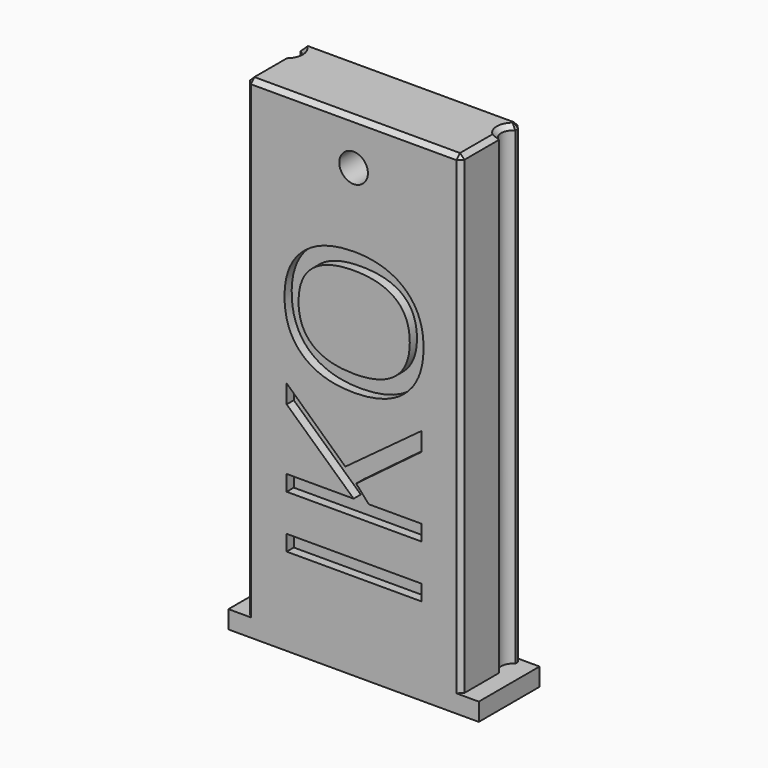
from build123d import *

# Parameters (mm, degrees)
F0_W         = 28
F0_H         = 8.5
F1_DEPTH     = 2
F3_DEPTH     = 53
F4_R         = 1.6
F5_DEPTH     = 8.501
F6_SIZE      = 0.5
F7_TEXT_SIZE = 21.1529840228
F8_DEPTH     = 1


# Not quite as in the source:
# - Text() gives the source's letters only with a copy of the font that has no kerning and outlines rounded to 1/6400 em; it was checked with that copy


with BuildPart() as f1:
    # F0 (on Top) → F1 (new body)
    with BuildSketch(Plane.XY):
        Rectangle(F0_W, F0_H)
    extrude(amount=F1_DEPTH)

    # F2 (on face) → F3 (join)
    with BuildSketch(Plane.XY.offset(2)):
        with BuildLine():
            Line((12, 4.25), (-12, 4.25))
            Line((-12, 4.25), (-12, 3.35))
            ThreePointArc((-12, 3.35), (-11.35, 2.2), (-12, 1.05))
            Line((-12, 1.05), (-12, -4.25))
            Line((-12, -4.25), (12, -4.25))
            Line((12, -4.25), (12, 1.05))
            ThreePointArc((12, 1.05), (11.35, 2.2), (12, 3.35))
            Line((12, 3.35), (12, 4.25))
        make_face()
    extrude(amount=F3_DEPTH)

    # F4 (on face) → F5 (cut, through all)
    with BuildSketch(Plane(origin=(0, 4.25, 0), x_dir=(-1, 0, 0), z_dir=(0, 1, 0))):
        with Locations((0, 50)):
            Circle(F4_R)
    extrude(amount=-F5_DEPTH, mode=Mode.SUBTRACT)

    # F6
    f6_edges = [f1.edges().sort_by_distance(p)[0] for p in [
        (12, 3.8, 55),
        (0, 4.25, 55),
        (-12, 3.8, 55),
        (-11.35, 2.2, 55),
        (-12, -1.6, 55),
        (0, -4.25, 55),
        (12, -1.6, 55),
        (11.35, 2.2, 55),
        (-12, 4.25, 28.5),
        (12, 4.25, 28.5),
        (-12, -4.25, 28.5),
        (12, -4.25, 28.5),
    ]]
    chamfer(f6_edges, length=F6_SIZE)

    # F7 (on face) → F8 (cut)
    with BuildSketch(Plane.XZ.offset(4.25)):
        with Locations(Location((7.6150742482, 7.7036715641), (0, 0, 90))):
            Text('IKO', F7_TEXT_SIZE, font='Open Sans', text_align=(TextAlign.LEFT, TextAlign.BOTTOM))
    extrude(amount=-F8_DEPTH, mode=Mode.SUBTRACT)


solid = f1.part
